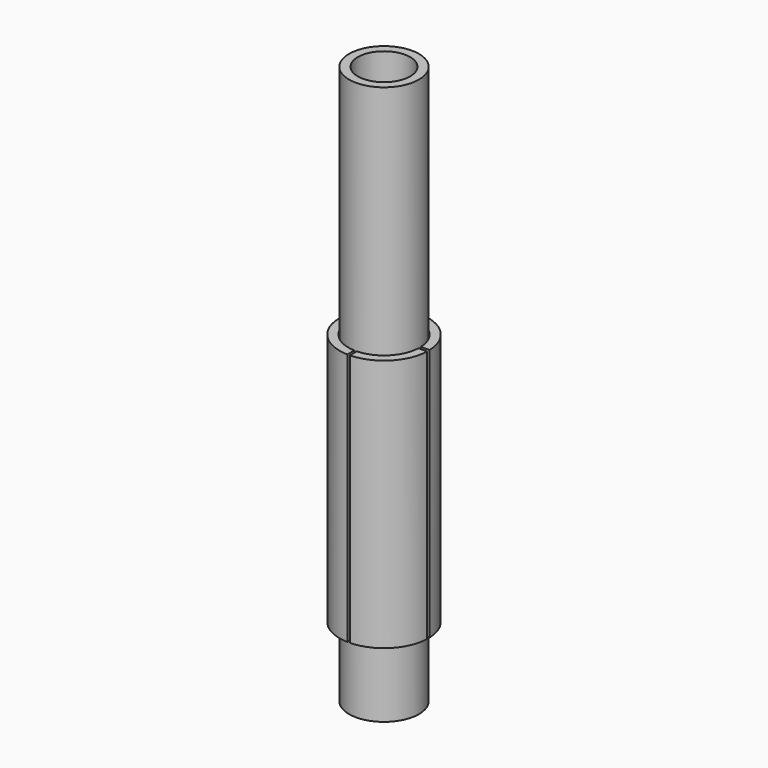
from build123d import *

# Parameters (mm, degrees)
F0_R     = 12.7
F0_R_2   = 9.525
F1_DEPTH = 177.8
F2_R     = 16.129
F2_R_2   = 12.954
F3_DEPTH = 92.075
F4_W     = 3.7774993107
F4_H     = 1.0993301403
F5_DEPTH = 177.801
F6_W     = 3.6055315286
F6_H     = 0.8748579712
F6_W_2   = 0.9862377919
F6_H_2   = 3.7802174482
F7_DEPTH = 92.075
F8_DEPTH = 25.4


# Not quite as in the source:
# - a feature names something its author has since deleted; it is built from what else it names


with BuildPart() as f1:
    # F0 (on Top) → F1 (new body)
    with BuildSketch(Plane.XY):
        Circle(F0_R)
        Circle(F0_R_2, mode=Mode.SUBTRACT)
    extrude(amount=F1_DEPTH)

    # F8 (add): a face of the model
    f8_faces = [f1.faces().sort_by_distance(p)[0] for p in [
        (-12.3407897552, 0, 0),
    ]]
    extrude(f8_faces, amount=F8_DEPTH)


with BuildPart() as f3:
    # F2 (on Top) → F3 (new body)
    with BuildSketch(Plane.XY):
        Circle(F2_R)
        Circle(F2_R_2, mode=Mode.SUBTRACT)
    extrude(amount=F3_DEPTH)

    # F4 (on Top) → F5 (cut, through all)
    with BuildSketch(Plane.XY):
        with Locations((14.8086710833, 0.0370488851)):
            Rectangle(F4_W, F4_H)
    extrude(amount=F5_DEPTH, mode=Mode.SUBTRACT)

    # F6 (on Top) → F7 (cut, through all)
    with BuildSketch(Plane.XY):
        with Locations((-14.6675733849, 0.0279923697)):
            Rectangle(F6_W, F6_H)
        Polygon((0.4868659598, -12.8129947375), (-0.4289262579, -12.8546217456), (-0.4289262579, -16.4708271623), (0.4868659598, -16.4708271623), align=None)
        with Locations((0.0407108382, 14.701657732)):
            Rectangle(F6_W_2, F6_H_2)
    extrude(amount=F7_DEPTH, mode=Mode.SUBTRACT)


solid = Compound([f1.part, f3.part])
